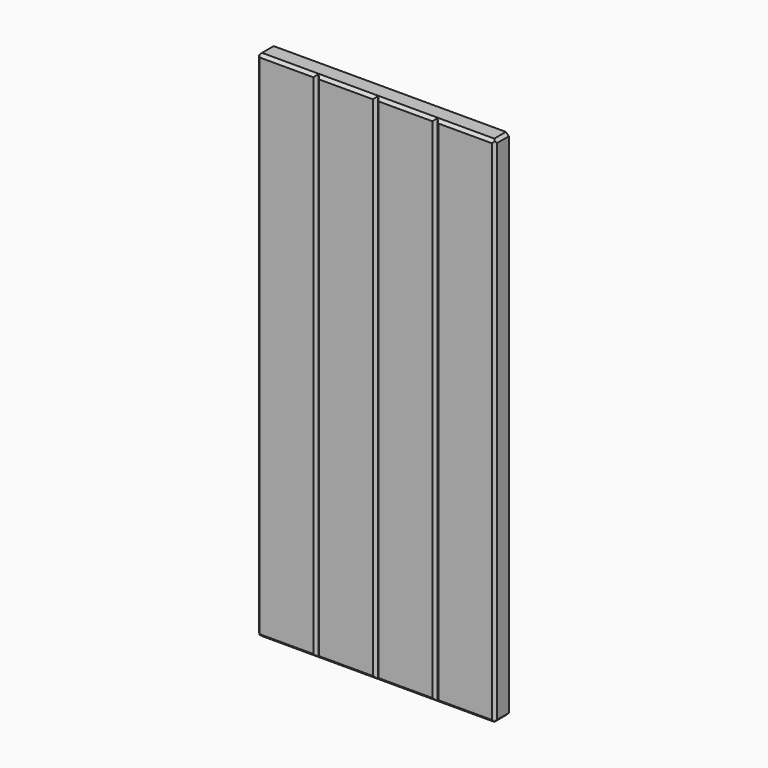
from build123d import *

# Parameters (mm, degrees)
F0_W       = 259.08
F0_H       = 558.8
F1_DEPTH   = 19.05
F3_DEPTH   = 558.801
F4_C1_SIZE = 3.175
F4_C2_SIZE = 3.175
F4_C3_SIZE = 3.175
F5_SIZE    = 3.175
F6_SIZE    = 3.175


# Not quite as in the source:
# - a feature names something its author has since deleted; it is built from what else it names


with BuildPart() as f1:
    # F0 (on Front) → F1 (new body)
    with BuildSketch(Plane.XZ):
        Rectangle(F0_W, F0_H)
    extrude(amount=F1_DEPTH)

    # F2 (on face) → F3 (cut, through all)
    with BuildSketch(Plane(origin=(0, 0, -279.4), x_dir=(1, 0, 0), z_dir=(0, 0, -1))):
        Polygon((-64.77, 19.05), (-67.945, 19.05), (-64.77, 16.0336531699), (-61.595, 19.05), align=None)
        Polygon((0, 16.0336531699), (3.175, 19.05), (0, 19.05), (-3.175, 19.05), align=None)
        Polygon((64.77, 16.0336531699), (67.945, 19.05), (64.77, 19.05), (61.595, 19.05), align=None)
    extrude(amount=-F3_DEPTH, mode=Mode.SUBTRACT)

    # F4: chamfer of 3.175 on 4 edges, made by hand

    # F4_c1
    f4_c1_edges = [f1.edges().sort_by_distance(p)[0] for p in [
        (-98.7425, -19.05, -279.4),
    ]]
    chamfer(f4_c1_edges, length=F4_C1_SIZE)

    # F4_c2
    f4_c2_edges = [f1.edges().sort_by_distance(p)[0] for p in [
        (-98.7425, -19.05, 279.4),
    ]]
    chamfer(f4_c2_edges, length=F4_C2_SIZE)

    # F4_c3
    f4_c3_edges = [f1.edges().sort_by_distance(p)[0] for p in [
        (-129.54, -19.05, 0),
    ]]
    chamfer(f4_c3_edges, length=F4_C3_SIZE)

    # F5
    f5_edges = [f1.edges().sort_by_distance(p)[0] for p in [
        (-129.54, -7.9375, 279.4),
        (129.54, -7.9375, 279.4),
        (129.54, -7.9375, -279.4),
        (-129.54, -7.9375, -279.4),
    ]]
    chamfer(f5_edges, length=F5_SIZE)

    # F6
    f6_edges = [f1.edges().sort_by_distance(p)[0] for p in [
        (129.54, -19.05, 0),
    ]]
    chamfer(f6_edges, length=F6_SIZE)


solid = f1.part
